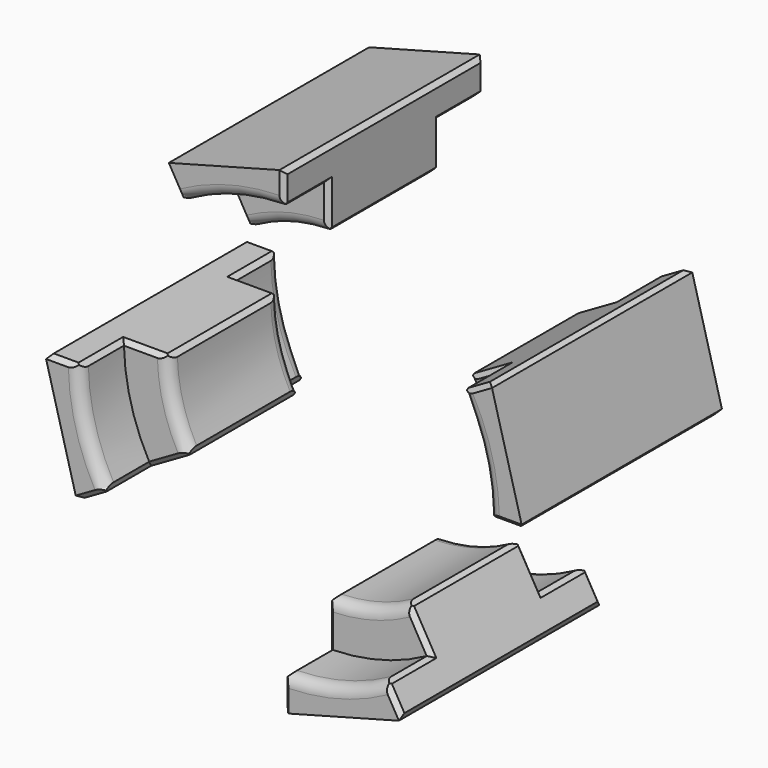
from build123d import *

# Parameters (mm, degrees)
F1_DEPTH     = 22.5
F3_DEPTH     = 12.5
F4_T1_DEPTH  = 12.1146927807
F4_T3_DEPTH  = 49.1876443864
F4_T5_DEPTH  = 12.0366296356
F4_T7_DEPTH  = 29.0620360822
F4_T9_DEPTH  = 12.0366296356
F4_T11_DEPTH = 12.1146927807
F4_T16_DEPTH = 12.1146927807
F4_S17_R     = 36.75
F4_T18_DEPTH = 8
F4_T22_DEPTH = 12.1146927807
F4_S23_R     = 36.75
F4_T24_DEPTH = 8
F4_T28_DEPTH = 12.1146927807
F4_S29_R     = 36.75
F4_T30_DEPTH = 8
F4_T34_DEPTH = 12.1146927807
F4_S35_R     = 36.75
F4_T36_DEPTH = 8
F4_T41_DEPTH = 12.0366296356
F4_T45_DEPTH = 12.1146927807
F4_S46_R     = 36.75
F4_T47_DEPTH = 8
F4_T53_DEPTH = 12.1146927807
F4_S54_R     = 36.75
F4_T55_DEPTH = 8
F4_T58_DEPTH = 12.0366296356
F4_T65_DEPTH = 12.0366296356
F4_T69_DEPTH = 12.1146927807
F4_S70_R     = 36.75
F4_T71_DEPTH = 8
F4_T77_DEPTH = 12.0366296356
F4_T81_DEPTH = 12.1146927807
F4_S82_R     = 36.75
F4_T83_DEPTH = 8
F5_R         = 2
F8_DEPTH     = 45.0010001
F9_COUNT     = 4


# Not quite as in the source:
# - a fillet or chamfer that OpenCascade refuses, or shapes differently, is made with other operations: its cross-section is extruded or revolved along the edge and cut away or added


with BuildPart() as f1:
    # F0 (on Front) → F1 (new body, symmetric)
    with BuildSketch(Plane.XZ):
        with BuildLine():
            Line((38.7546368194, 22.375), (31.8264335891, 18.375))
            ThreePointArc((31.8264335891, 18.375), (35.4977741161, 9.5115999075), (36.75, 0))
            Line((36.75, 0), (44.75, 0))
            ThreePointArc((44.75, 0), (43.2251807264, 11.5821522683), (38.7546368194, 22.375))
        make_face()
    extrude(amount=F1_DEPTH, both=True)

    # F2 (on Front) → F3 (join, symmetric)
    with BuildSketch(Plane.XZ):
        with BuildLine():
            Line((28.75, 0), (36.75, 0))
            ThreePointArc((36.75, 0), (35.4977741161, 9.5115999075), (31.8264335891, 18.375))
            Line((31.8264335891, 18.375), (24.8982303588, 14.375))
            ThreePointArc((24.8982303588, 14.375), (27.7703675058, 7.4410475467), (28.75, 0))
        make_face()
    extrude(amount=F3_DEPTH, both=True)

    # F4: chamfer of 0.8 on 16 edges, made by hand

    # F4_s2 → F4_t1 (cut)
    with BuildSketch(Plane.YZ.offset(34.6926536096)):
        Polygon((21.7, 0), (22.5, 0.8), (22.5, 0), align=None)
        Polygon((-21.7, 0), (-22.5, 0.8), (-22.5, 0), align=None)
    extrude(amount=F4_T1_DEPTH, mode=Mode.SUBTRACT)

    # F4_s4 → F4_t3 (cut)
    with BuildSketch(Plane.XZ.offset(-24.5938221932)):
        with BuildLine():
            Line((43.9427183957, 0), (44.7425858522, 0.8145620023))
            ThreePointArc((44.7425858522, 0.8145620023), (44.7480420438, 0.4186087071), (44.75, 0))
            Line((44.75, 0), (43.9427183957, 0))
        make_face()
        with BuildLine():
            Line((39.1554969802, 21.6658615392), (38.055510442, 21.9713591978))
            Line((38.055510442, 21.9713591978), (38.7546368194, 22.375))
            ThreePointArc((38.7546368194, 22.375), (38.9622455331, 22.0114952473), (39.1554969802, 21.6658615392))
        make_face()
    extrude(amount=F4_T3_DEPTH, mode=Mode.SUBTRACT)

    # F4_s6 → F4_t5 (cut)
    with BuildSketch(Plane.XZ.offset(12.5)):
        with BuildLine():
            Line((37.541477062, 0), (36.7416586426, 0.7829560586))
            ThreePointArc((36.7416586426, 0.7829560586), (36.7477922892, 0.4028174188), (36.75, 0))
            Line((36.75, 0), (37.541477062, 0))
        make_face()
        with BuildLine():
            Line((32.210687791, 17.6927694845), (32.5118728313, 18.770738531))
            Line((32.5118728313, 18.770738531), (31.8264335891, 18.375))
            ThreePointArc((31.8264335891, 18.375), (32.0259303648, 18.0250460268), (32.210687791, 17.6927694845))
        make_face()
    extrude(amount=F4_T5_DEPTH, mode=Mode.SUBTRACT)

    # F4_s8 → F4_t7 (cut)
    with BuildSketch(Plane.XZ.offset(-14.5310180411)):
        with BuildLine():
            Line((29.5391689118, 0), (28.7394621392, 0.7783417936))
            ThreePointArc((28.7394621392, 0.7783417936), (28.747209951, 0.4005246946), (28.75, 0))
            Line((28.75, 0), (29.5391689118, 0))
        make_face()
        with BuildLine():
            Line((25.5816706843, 14.7695844559), (25.2782752005, 13.6956673036))
            ThreePointArc((25.2782752005, 13.6956673036), (25.0960764528, 14.0267404152), (24.8982303588, 14.375))
            Line((24.8982303588, 14.375), (25.5816706843, 14.7695844559))
        make_face()
    extrude(amount=F4_T7_DEPTH, mode=Mode.SUBTRACT)

    # F4_s10 → F4_t9 (cut)
    with BuildSketch(Plane.XZ.offset(-24.5366296356)):
        with BuildLine():
            Line((37.541477062, 0), (36.7416586426, 0.7829560586))
            ThreePointArc((36.7416586426, 0.7829560586), (36.7477922892, 0.4028174188), (36.75, 0))
            Line((36.75, 0), (37.541477062, 0))
        make_face()
        with BuildLine():
            Line((32.210687791, 17.6927694845), (32.5118728313, 18.770738531))
            Line((32.5118728313, 18.770738531), (31.8264335891, 18.375))
            ThreePointArc((31.8264335891, 18.375), (32.0259303648, 18.0250460268), (32.210687791, 17.6927694845))
        make_face()
    extrude(amount=F4_T9_DEPTH, mode=Mode.SUBTRACT)

    # F4_s12 → F4_t11 (cut)
    with BuildSketch(Plane(origin=(40.5363510578, 0, 23.4036731952), x_dir=(0, 1, 0), z_dir=(-0.8660254038, 0, -0.5))):
        Polygon((22.5, 0.8), (21.7, 0), (22.5, 0), align=None)
        Polygon((-22.5, 0.8), (-21.7, 0), (-22.5, 0), align=None)
    extrude(amount=F4_T11_DEPTH, mode=Mode.SUBTRACT)


with BuildPart() as f4_tool14:
    # F4_s15 → F4_t16 (new body)
    with BuildSketch(Plane.YZ.offset(26.6926536096)):
        Polygon((-11.7, 0), (-12.5, 0.8), (-12.5, 0), align=None)
    extrude(amount=F4_T16_DEPTH)

    # F4_s17 → F4_t18 (intersect, symmetric)
    with BuildSketch(Plane.XZ.offset(12.1)):
        Circle(F4_S17_R)
    extrude(amount=F4_T18_DEPTH, both=True, mode=Mode.INTERSECT)


with BuildPart() as f1_1:
    add(f1.part)

    # F4_t13: cut F4_tool14
    add(f4_tool14.part, mode=Mode.SUBTRACT)


with BuildPart() as f4_tool20:
    # F4_s21 → F4_t22 (new body)
    with BuildSketch(Plane.YZ.offset(26.6926536096)):
        Polygon((11.7, 0), (12.5, 0.8), (12.5, 0), align=None)
    extrude(amount=F4_T22_DEPTH)

    # F4_s23 → F4_t24 (intersect, symmetric)
    with BuildSketch(Plane.XZ.offset(-12.1)):
        Circle(F4_S23_R)
    extrude(amount=F4_T24_DEPTH, both=True, mode=Mode.INTERSECT)


with BuildPart() as f1_2:
    add(f1_1.part)

    # F4_t19: cut F4_tool20
    add(f4_tool20.part, mode=Mode.SUBTRACT)


with BuildPart() as f4_tool26:
    # F4_s27 → F4_t28 (new body)
    with BuildSketch(Plane(origin=(33.6081478275, 0, 19.4036731952), x_dir=(0, 1, 0), z_dir=(-0.8660254038, 0, -0.5))):
        Polygon((11.7, 0), (12.5, 0.8), (12.5, 0), align=None)
    extrude(amount=F4_T28_DEPTH)

    # F4_s29 → F4_t30 (intersect, symmetric)
    with BuildSketch(Plane.XZ.offset(-12.1)):
        Circle(F4_S29_R)
    extrude(amount=F4_T30_DEPTH, both=True, mode=Mode.INTERSECT)


with BuildPart() as f1_3:
    add(f1_2.part)

    # F4_t25: cut F4_tool26
    add(f4_tool26.part, mode=Mode.SUBTRACT)


with BuildPart() as f4_tool32:
    # F4_s33 → F4_t34 (new body)
    with BuildSketch(Plane(origin=(33.6081478275, 0, 19.4036731952), x_dir=(0, 1, 0), z_dir=(-0.8660254038, 0, -0.5))):
        Polygon((-11.7, 0), (-12.5, 0.8), (-12.5, 0), align=None)
    extrude(amount=F4_T34_DEPTH)

    # F4_s35 → F4_t36 (intersect, symmetric)
    with BuildSketch(Plane.XZ.offset(12.1)):
        Circle(F4_S35_R)
    extrude(amount=F4_T36_DEPTH, both=True, mode=Mode.INTERSECT)


with BuildPart() as f1_4:
    add(f1_3.part)

    # F4_t31: cut F4_tool32
    add(f4_tool32.part, mode=Mode.SUBTRACT)


with BuildPart() as f4_tool39:
    # F4_s40 → F4_t41 (new body)
    with BuildSketch(Plane.XZ.offset(22.5)):
        with BuildLine():
            Line((37.541477062, 0), (36.7416586426, 0.7829560586))
            ThreePointArc((36.7416586426, 0.7829560586), (36.7477922892, 0.4028174188), (36.75, 0))
            Line((36.75, 0), (37.541477062, 0))
        make_face()
    extrude(amount=-F4_T41_DEPTH)

    split(bisect_by=Plane.XZ.offset(12.5), keep=Keep.BOTTOM)


with BuildPart() as f4_tool43:
    # F4_s44 → F4_t45 (new body)
    with BuildSketch(Plane.YZ.offset(26.6926536096)):
        Polygon((-11.7, 0), (-12.5, 0.8), (-12.5, 0), align=None)
    extrude(amount=F4_T45_DEPTH)

    # F4_s46 → F4_t47 (cut, symmetric)
    with BuildSketch(Plane.XZ.offset(12.1)):
        Circle(F4_S46_R)
    extrude(amount=F4_T47_DEPTH, both=True, mode=Mode.SUBTRACT)


with BuildPart() as f4_tool39_1:
    add(f4_tool39.part)

    # F4_t48: intersect F4_tool43
    add(f4_tool43.part, mode=Mode.INTERSECT)


with BuildPart() as f1_5:
    add(f1_4.part)

    # F4_t37: cut F4_tool39
    add(f4_tool39_1.part, mode=Mode.SUBTRACT)


with BuildPart() as f4_tool51:
    # F4_s52 → F4_t53 (new body)
    with BuildSketch(Plane.YZ.offset(26.6926536096)):
        Polygon((11.7, 0), (12.5, 0.8), (12.5, 0), align=None)
    extrude(amount=F4_T53_DEPTH)

    # F4_s54 → F4_t55 (cut, symmetric)
    with BuildSketch(Plane.XZ.offset(-12.1)):
        Circle(F4_S54_R)
    extrude(amount=F4_T55_DEPTH, both=True, mode=Mode.SUBTRACT)


with BuildPart() as f4_tool56:
    # F4_s57 → F4_t58 (new body)
    with BuildSketch(Plane.XZ.offset(-10.4633703644)):
        with BuildLine():
            Line((37.541477062, 0), (36.7416586426, 0.7829560586))
            ThreePointArc((36.7416586426, 0.7829560586), (36.7477922892, 0.4028174188), (36.75, 0))
            Line((36.75, 0), (37.541477062, 0))
        make_face()
    extrude(amount=-F4_T58_DEPTH)

    split(bisect_by=Plane.XZ.offset(-12.5), keep=Keep.TOP)


with BuildPart() as f4_tool51_1:
    add(f4_tool51.part)

    # F4_t60: intersect F4_tool56
    add(f4_tool56.part, mode=Mode.INTERSECT)


with BuildPart() as f1_6:
    add(f1_5.part)

    # F4_t49: cut F4_tool51
    add(f4_tool51_1.part, mode=Mode.SUBTRACT)


with BuildPart() as f4_tool63:
    # F4_s64 → F4_t65 (new body)
    with BuildSketch(Plane.XZ.offset(-10.4633703644)):
        with BuildLine():
            Line((32.210687791, 17.6927694845), (32.5118728313, 18.770738531))
            Line((32.5118728313, 18.770738531), (31.8264335891, 18.375))
            ThreePointArc((31.8264335891, 18.375), (32.0259303648, 18.0250460268), (32.210687791, 17.6927694845))
        make_face()
    extrude(amount=-F4_T65_DEPTH)

    split(bisect_by=Plane.XZ.offset(-12.5), keep=Keep.TOP)


with BuildPart() as f4_tool67:
    # F4_s68 → F4_t69 (new body)
    with BuildSketch(Plane(origin=(33.6081478275, 0, 19.4036731952), x_dir=(0, 1, 0), z_dir=(-0.8660254038, 0, -0.5))):
        Polygon((11.7, 0), (12.5, 0.8), (12.5, 0), align=None)
    extrude(amount=F4_T69_DEPTH)

    # F4_s70 → F4_t71 (cut, symmetric)
    with BuildSketch(Plane.XZ.offset(-12.1)):
        Circle(F4_S70_R)
    extrude(amount=F4_T71_DEPTH, both=True, mode=Mode.SUBTRACT)


with BuildPart() as f4_tool63_1:
    add(f4_tool63.part)

    # F4_t72: intersect F4_tool67
    add(f4_tool67.part, mode=Mode.INTERSECT)


with BuildPart() as f1_7:
    add(f1_6.part)

    # F4_t61: cut F4_tool63
    add(f4_tool63_1.part, mode=Mode.SUBTRACT)


with BuildPart() as f4_tool75:
    # F4_s76 → F4_t77 (new body)
    with BuildSketch(Plane.XZ.offset(22.5)):
        with BuildLine():
            Line((32.210687791, 17.6927694845), (32.5118728313, 18.770738531))
            Line((32.5118728313, 18.770738531), (31.8264335891, 18.375))
            ThreePointArc((31.8264335891, 18.375), (32.0259303648, 18.0250460268), (32.210687791, 17.6927694845))
        make_face()
    extrude(amount=-F4_T77_DEPTH)

    split(bisect_by=Plane.XZ.offset(12.5), keep=Keep.BOTTOM)


with BuildPart() as f4_tool79:
    # F4_s80 → F4_t81 (new body)
    with BuildSketch(Plane(origin=(33.6081478275, 0, 19.4036731952), x_dir=(0, 1, 0), z_dir=(-0.8660254038, 0, -0.5))):
        Polygon((-11.7, 0), (-12.5, 0.8), (-12.5, 0), align=None)
    extrude(amount=F4_T81_DEPTH)

    # F4_s82 → F4_t83 (cut, symmetric)
    with BuildSketch(Plane.XZ.offset(12.1)):
        Circle(F4_S82_R)
    extrude(amount=F4_T83_DEPTH, both=True, mode=Mode.SUBTRACT)


with BuildPart() as f4_tool75_1:
    add(f4_tool75.part)

    # F4_t84: intersect F4_tool79
    add(f4_tool79.part, mode=Mode.INTERSECT)


with BuildPart() as f1_8:
    add(f1_7.part)

    # F4_t73: cut F4_tool75
    add(f4_tool75_1.part, mode=Mode.SUBTRACT)

    # F5
    f5_edges = [f1_8.edges().sort_by_distance(p)[0] for p in [
        (27.770368, -12.5, 7.441048),
        (35.497774, -22.5, 9.5116),
        (43.225181, -22.5, 11.582152),
        (43.225181, 22.5, 11.582152),
        (35.497774, 22.5, 9.5116),
        (27.770368, 12.5, 7.441048),
    ]]
    fillet(f5_edges, radius=F5_R)

    # F7 (on face) → F8 (cut, through all)
    with BuildSketch(Plane.XZ.offset(22.5)):
        Polygon((34.7195765394, 21.6289372416), (37.4161029148, 20.6784366592), (42.7425139644, 0.8), (37.5549691263, -4.785540048), (62.7318742219, 6.0370126739), (46.87034473, 30.1799183012), align=None)
    extrude(amount=-F8_DEPTH, mode=Mode.SUBTRACT)


with BuildPart() as f9_1:
    # F9: instance of F1
    add(f1_8.part.rotate(Axis((0, 0, 0), (0, 1, 0)), 1 * 360 / F9_COUNT))


with BuildPart() as f9_2:
    # F9: instance of F1
    add(f1_8.part.rotate(Axis((0, 0, 0), (0, 1, 0)), 2 * 360 / F9_COUNT))


with BuildPart() as f9_3:
    # F9: instance of F1
    add(f1_8.part.rotate(Axis((0, 0, 0), (0, 1, 0)), 3 * 360 / F9_COUNT))


solid = Compound([f1_8.part, f9_1.part, f9_2.part, f9_3.part])
